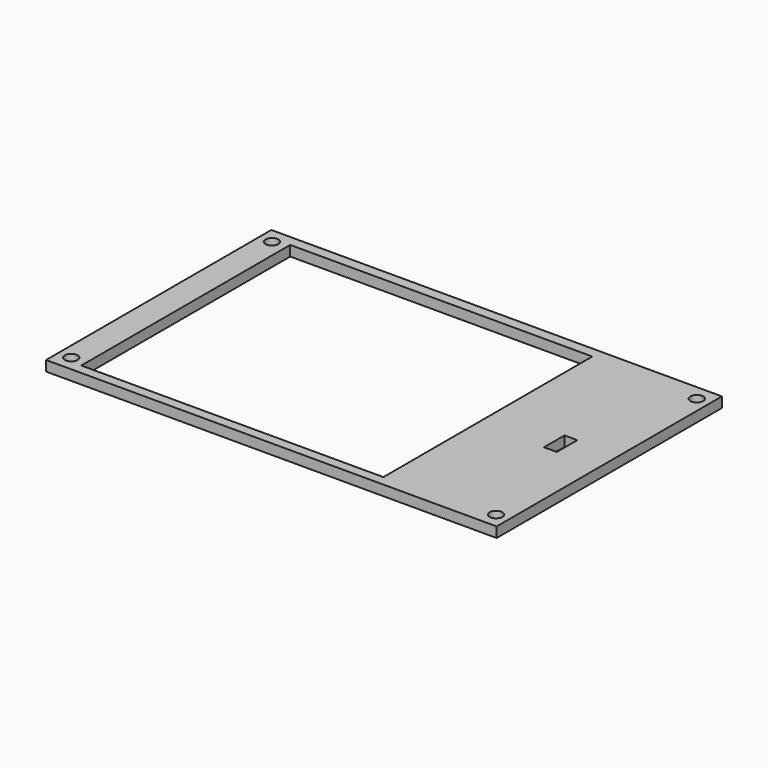
from build123d import *

# Parameters (mm, degrees)
F0_R     = 3.175
F1_DEPTH = 5.08


# Not quite as in the source:
# - a feature names something its author has since deleted; it is built from what else it names


with BuildPart() as f1:
    # F0 (on Top) → F1 (new body)
    with BuildSketch(Plane.XY):
        Polygon((-196.7800016522, 116.4700038791), (-196.7814051471, 116.4700038791), (-202.7097940445, 116.4700038791), (-202.7097940445, 108.8500038791), (-202.7097940445, 101.2300038791), (-202.7097940445, -23.2299961209), (-196.7800016522, -23.2299961209), (20.8102059555, -23.2299961209), (20.8102059555, 116.4700038791), (15.3085948529, 116.4700038791), (-35.4914051471, 116.4700038791), (-39.3014051471, 116.4700038791), (-90.9497940445, 116.4700038791), (-187.4697940445, 116.4700038791), (-189.1614051471, 116.4700038791), (-195.0897940445, 116.4700038791), align=None)
        with Locations((-196.3344303894, -15.6099961209)):
            Circle(F0_R, mode=Mode.SUBTRACT)
        Polygon((-189.1614051471, -18.3182691255), (-189.1614051471, 111.2217308745), (-189.1583133745, 111.2217308745), (-39.3014051471, 111.2217308745), (-39.3014051471, -18.3182691255), align=None, mode=Mode.SUBTRACT)
        with Locations((14.4348423004, -15.6099961209)):
            Circle(F0_R, mode=Mode.SUBTRACT)
        Polygon((0, 52.8017308745), (0, 46.4517308745), (0, 40.1017308745), (-6.35, 40.1017308745), (-6.35, 46.4517308745), (-6.35, 52.8017308745), align=None, mode=Mode.SUBTRACT)
        with Locations((-196.3344303894, 108.8500038791)):
            Circle(F0_R, mode=Mode.SUBTRACT)
        with Locations((14.4348423004, 108.8500038791)):
            Circle(F0_R, mode=Mode.SUBTRACT)
    extrude(amount=F1_DEPTH)


solid = f1.part
